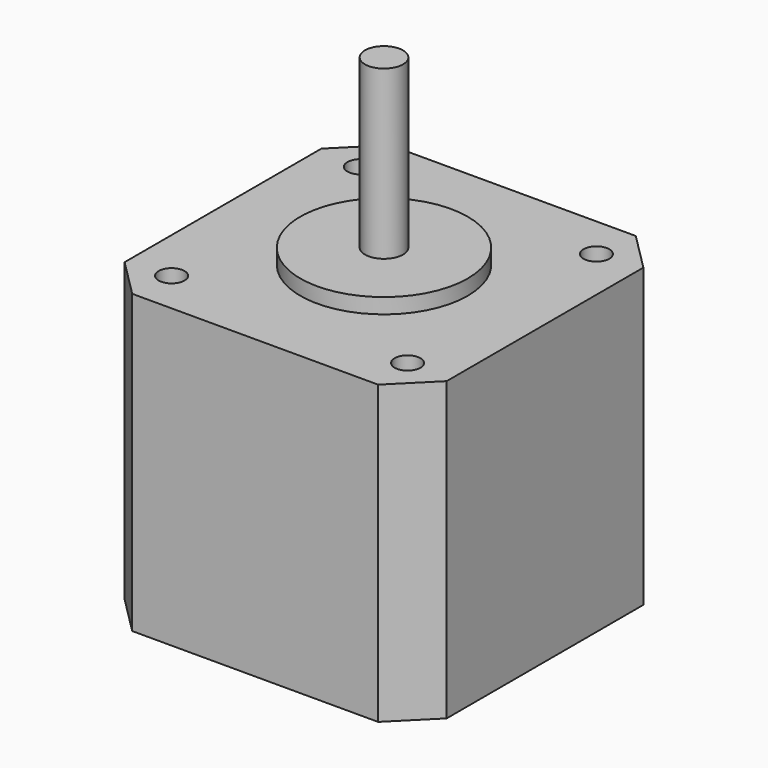
from build123d import *

# Parameters (mm, degrees)
F0_W     = 42.3
F0_H     = 42.3
F1_DEPTH = 39
F2_R     = 2.5
F3_DEPTH = 24
F2_R_2   = 11
F4_DEPTH = 2
F5_D     = 3.4
F5_DEPTH = 12
F5_TIP   = 1.0214630523
F6_SIZE  = 5


with BuildPart() as f1:
    # F0 (on Top) → F1 (new body)
    with BuildSketch(Plane.XY):
        Rectangle(F0_W, F0_H)
    extrude(amount=-F1_DEPTH)

    # F2 (on face) → F4 (join)
    with BuildSketch(Plane.XY):
        Circle(F2_R_2)
        Circle(F2_R, mode=Mode.SUBTRACT)
    extrude(amount=F4_DEPTH)

    # F5
    with Locations(Plane.XY):
        with Locations((15.5, -15.5), (15.5, 15.5), (-15.5, -15.5), (-15.5, 15.5)):
            Hole(F5_D / 2, depth=F5_DEPTH)
            with Locations((0, 0, -(F5_DEPTH + F5_TIP / 2))):  # 118° drill point
                Cone(0, F5_D / 2, F5_TIP, mode=Mode.SUBTRACT)

    # F6
    f6_edges = [f1.edges().sort_by_distance(p)[0] for p in [
        (-21.15, -21.15, -19.5),
        (21.15, 21.15, -19.5),
        (21.15, -21.15, -19.5),
        (-21.15, 21.15, -19.5),
    ]]
    chamfer(f6_edges, length=F6_SIZE)


with BuildPart() as f3:
    # F2 (on face) → F3 (new body)
    with BuildSketch(Plane.XY):
        Circle(F2_R)
    extrude(amount=F3_DEPTH)


solid = Compound([f1.part, f3.part])
